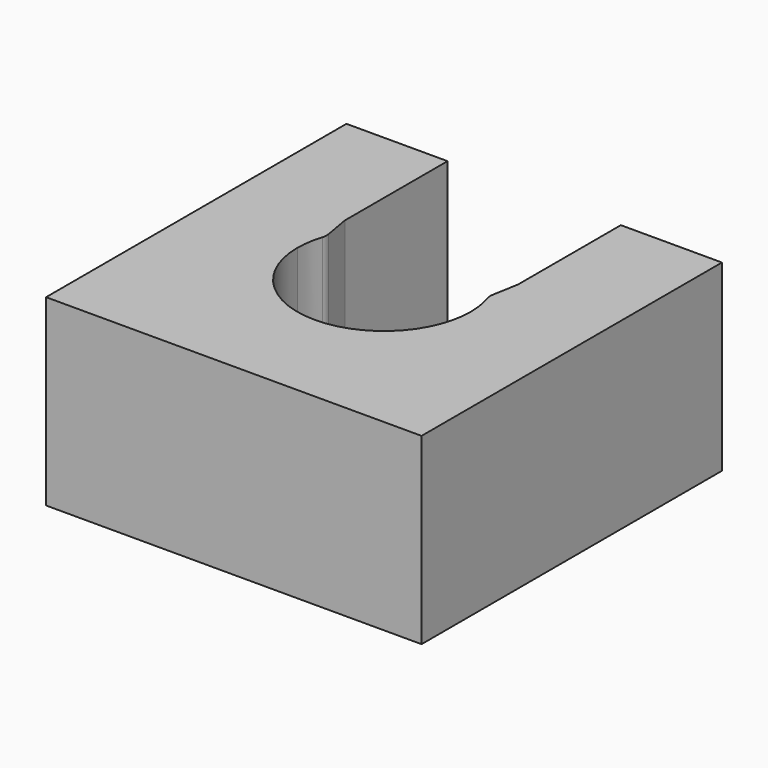
from build123d import *

# Parameters (mm, degrees)
F1_DEPTH = 12.7


# Not quite as in the source:
# - a length typed as a fraction of an inch, garbled in the dataset ("3 / 203.2 mm" for 3/8 in), is restored


with BuildPart() as f1:
    # F0 (on Top) → F1 (new body)
    with BuildSketch(Plane.XY):
        with BuildLine():
            Line((-6, 13), (-13, 13))
            Line((-13, 13), (-13, -13))
            Line((-13, -13), (13, -13))
            Line((13, -13), (13, 13))
            Line((13, 13), (6, 13))
            Line((6, 13), (6, 4.1042417199))
            Line((6, 4.1042417199), (5.6827738736, 2.3051629565))
            ThreePointArc((5.6827738736, 2.3051629565), (5.6698549343, 2.0641245171), (5.7150699657, 1.8270126676))
            ThreePointArc((5.7150699657, 1.8270126676), (5.9283395565, 0.9245485942), (6, 0))
            ThreePointArc((6, 0), (0, -6), (-6, 0))
            ThreePointArc((-6, 0), (-5.9283395565, 0.9245485942), (-5.7150699657, 1.8270126676))
            ThreePointArc((-5.7150699657, 1.8270126676), (-5.6698549343, 2.0641245171), (-5.6827738736, 2.3051629565))
            Line((-5.6827738736, 2.3051629565), (-6, 4.1042417199))
            Line((-6, 4.1042417199), (-6, 13))
        make_face()
    extrude(amount=F1_DEPTH)


solid = f1.part
